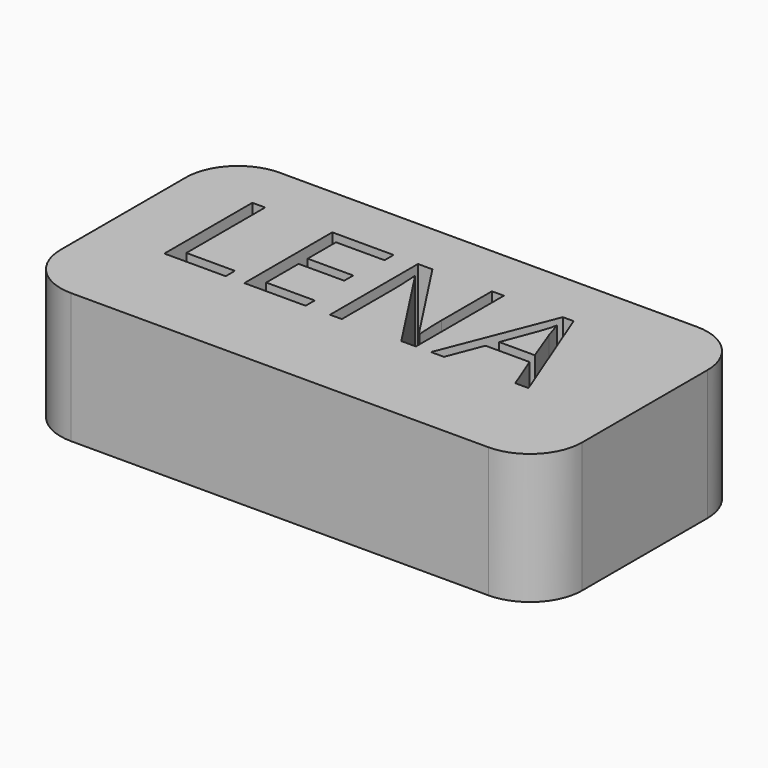
from build123d import *

# Parameters (mm, degrees)
F0_W         = 50.8
F0_H         = 25.4
F1_DEPTH     = 12.7
F2_R         = 5.08
F3_TEXT_SIZE = 15.0057911505
F4_DEPTH     = 25.4


# Not quite as in the source:
# - Text() gives the source's letters only with a copy of the font that has no kerning and outlines rounded to 1/6400 em; it was checked with that copy


with BuildPart() as f1:
    # F0 (on Top) → F1 (new body)
    with BuildSketch(Plane.XY):
        with Locations((25.4, 12.7)):
            Rectangle(F0_W, F0_H)
    extrude(amount=F1_DEPTH)

    # F2
    f2_edges = [f1.edges().sort_by_distance(p)[0] for p in [
        (0, 0, 6.35),
        (50.8, 0, 6.35),
        (50.8, 25.4, 6.35),
        (0, 25.4, 6.35),
    ]]
    fillet(f2_edges, radius=F2_R)

    # F3 (on face) → F4 (cut)
    with BuildSketch(Plane.XY.offset(12.7)):
        with Locations((5.08, 9.5158303716)):
            Text('LENA', F3_TEXT_SIZE, font='Open Sans', text_align=(TextAlign.LEFT, TextAlign.BOTTOM))
    extrude(amount=-F4_DEPTH, mode=Mode.SUBTRACT)


solid = f1.part
